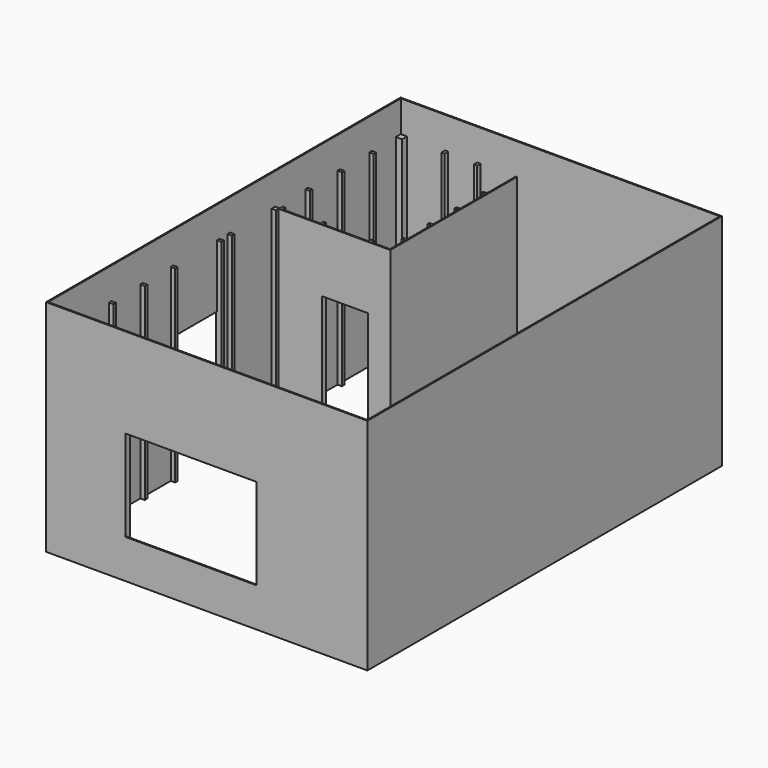
from build123d import *

# Parameters (mm, degrees)
F4_DEPTH  = 3500
F6_DEPTH  = 3000
F2_W      = 70
F2_H      = 50
F2_W_2    = 100
F2_H_2    = 100
F2_W_3    = 50
F2_H_3    = 70
F2_W_4    = 60
F2_H_4    = 40
F2_W_5    = 40
F2_H_5    = 60
F7_DEPTH  = 3000
F8_W      = 2086
F8_H      = 1450
F9_DEPTH  = 18
F10_W     = 869
F10_H     = 2000
F11_DEPTH = 18
F12_W     = 727
F12_H     = 2000
F13_DEPTH = 18


# Not quite as in the source:
# - a feature names something its author has since deleted; it is built from what else it names


with BuildPart() as f4:
    # F3 (on face) → F4 (new body)
    with BuildSketch(Plane.XY):
        Polygon((1830, 7038), (-18, 7038), (-18, 4500), (-18, -18), (5098, -18), (5098, 7038), align=None)
        Polygon((0, 4500), (0, 7020), (1830, 7020), (5080, 7020), (5080, 0), (0, 0), align=None, mode=Mode.SUBTRACT)
    extrude(amount=F4_DEPTH)

    # F5 (on face) → F6 (join)
    with BuildSketch(Plane.XY):
        Polygon((0, 4518), (0, 4500), (1830, 4500), (1848, 4500), (1848, 7020), (1830, 7020), (1830, 4518), align=None)
    extrude(amount=F6_DEPTH)

    # F2 (on Top) → F7 (join)
    with BuildSketch(Plane.XY):
        with Locations((35, 4475)):
            Rectangle(F2_W, F2_H)
        with Locations((35, 3600)):
            Rectangle(F2_W, F2_H)
        with Locations((35, 3385)):
            Rectangle(F2_W, F2_H)
        with Locations((35, 2466)):
            Rectangle(F2_W, F2_H)
        with Locations((35, 1861)):
            Rectangle(F2_W, F2_H)
        with Locations((35, 1236)):
            Rectangle(F2_W, F2_H)
        with Locations((35, 596)):
            Rectangle(F2_W, F2_H)
        with Locations((50, 50)):
            Rectangle(F2_W_2, F2_H_2)
        with Locations((652, 35)):
            Rectangle(F2_W_3, F2_H_3)
        with Locations((1224, 35)):
            Rectangle(F2_W_3, F2_H_3)
        with Locations((3360, 35)):
            Rectangle(F2_W_3, F2_H_3)
        with Locations((3830, 35)):
            Rectangle(F2_W_3, F2_H_3)
        with Locations((4425, 35)):
            Rectangle(F2_W_3, F2_H_3)
        with Locations((5045, 25)):
            Rectangle(F2_W, F2_H)
        with Locations((5045, 665)):
            Rectangle(F2_W, F2_H)
        with Locations((5045, 1305)):
            Rectangle(F2_W, F2_H)
        with Locations((5045, 1945)):
            Rectangle(F2_W, F2_H)
        with Locations((5045, 2585)):
            Rectangle(F2_W, F2_H)
        with Locations((5045, 3225)):
            Rectangle(F2_W, F2_H)
        with Locations((5045, 3865)):
            Rectangle(F2_W, F2_H)
        with Locations((5045, 4505)):
            Rectangle(F2_W, F2_H)
        with Locations((5045, 5145)):
            Rectangle(F2_W, F2_H)
        with Locations((5045, 5785)):
            Rectangle(F2_W, F2_H)
        with Locations((5045, 6425)):
            Rectangle(F2_W, F2_H)
        with Locations((50, 6970)):
            Rectangle(F2_W_2, F2_H_2)
        with Locations((729, 6985)):
            Rectangle(F2_W_3, F2_H_3)
        with Locations((1244, 6985)):
            Rectangle(F2_W_3, F2_H_3)
        with Locations((1800, 6428)):
            Rectangle(F2_W_4, F2_H_4)
        with Locations((1800, 5896)):
            Rectangle(F2_W_4, F2_H_4)
        with Locations((1800, 5354)):
            Rectangle(F2_W_4, F2_H_4)
        with Locations((1800, 4836)):
            Rectangle(F2_W_4, F2_H_4)
        with Locations((35, 6417)):
            Rectangle(F2_W, F2_H)
        with Locations((35, 5784)):
            Rectangle(F2_W, F2_H)
        with Locations((35, 5145)):
            Rectangle(F2_W, F2_H)
        with Locations((95, 4548)):
            Rectangle(F2_W_5, F2_H_5)
        with Locations((743, 4548)):
            Rectangle(F2_W_5, F2_H_5)
        with Locations((1510, 4548)):
            Rectangle(F2_W_5, F2_H_5)
    extrude(amount=F7_DEPTH)

    # F8 (on face) → F9 (cut, through all)
    with BuildSketch(Plane.XZ.offset(18)):
        with Locations((2292, 1345)):
            Rectangle(F8_W, F8_H)
    extrude(amount=-F9_DEPTH, mode=Mode.SUBTRACT)

    # F10 (on face) → F11 (cut, through all)
    with BuildSketch(Plane.YZ):
        with Locations((2925.5, 1000)):
            Rectangle(F10_W, F10_H)
    extrude(amount=-F11_DEPTH, mode=Mode.SUBTRACT)

    # F12 (on face) → F13 (cut, through all)
    with BuildSketch(Plane(origin=(0, 4518, 0), x_dir=(-1, 0, 0), z_dir=(0, 1, 0))):
        with Locations((-1126.5, 1000)):
            Rectangle(F12_W, F12_H)
    extrude(amount=-F13_DEPTH, mode=Mode.SUBTRACT)


solid = f4.part
